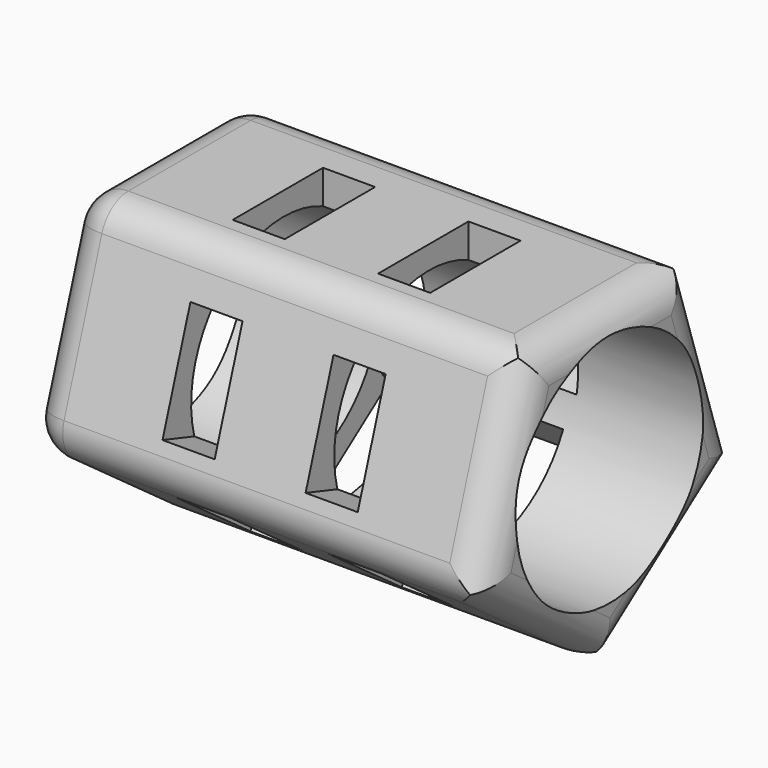
from build123d import *

# Parameters (mm, degrees)
F0_R         = 17.1087851354
F1_DEPTH     = 66.548
F2_T1_DEPTH  = 55.1463138897
F2_T3_DEPTH  = 55.1463138897
F2_T5_DEPTH  = 55.1463138897
F2_T7_DEPTH  = 55.1463138897
F2_T9_DEPTH  = 55.1463138897
F3_T1_DEPTH  = 22.3646418052
F3_T3_DEPTH  = 22.3646418052
F3_T5_DEPTH  = 22.3646418052
F3_T7_DEPTH  = 22.3646418052
F3_T9_DEPTH  = 22.3646418052
F3_T11_DEPTH = 65.6150901057
F3_T16_DEPTH = 5.1816
F3_T22_DEPTH = 5.1816
F3_T28_DEPTH = 5.1816
F3_T34_DEPTH = 5.1816
F3_T40_DEPTH = 5.1816
F4_W         = 7.62
F4_H         = 16.51
F5_DEPTH     = 7.874
F6_W         = 7.62
F6_H         = 16.51
F7_DEPTH     = 7.112
F8_W         = 7.62
F8_H         = 16.51
F9_DEPTH     = 12.192
F10_W        = 7.62
F10_H        = 16.51
F11_DEPTH    = 24.384
F12_W        = 7.62
F12_H        = 16.51
F13_DEPTH    = 25.4


# Not quite as in the source:
# - a fillet or chamfer that OpenCascade refuses, or shapes differently, is made with other operations: its cross-section is extruded or revolved along the edge and cut away or added


with BuildPart() as f1:
    # F0 (on Right) → F1 (new body)
    with BuildSketch(Plane.YZ):
        Polygon((14.8731569449, 20.4711443192), (-14.8731569449, 20.4711443192), (-24.0652734568, -7.8192813413), (0, -25.3037259558), (24.0652734568, -7.8192813413), align=None)
        Circle(F0_R, mode=Mode.SUBTRACT)
    extrude(amount=F1_DEPTH)

    # F2: fillet of radius 5.08 on 5 edges, made by hand

    # F2_s2 → F2_t1 (cut)
    with BuildSketch(Plane(origin=(0, 8.5205740845, 26.2236305872), x_dir=(1, 0, 0), z_dir=(0, -0.3090169944, -0.9510565163))):
        with BuildLine():
            ThreePointArc((61.468, 20.4711443192), (65.0601024484, 18.9832467676), (66.548, 15.3911443192))
            Line((66.548, 15.3911443192), (66.548, 20.4711443192))
            Line((66.548, 20.4711443192), (61.468, 20.4711443192))
        make_face()
    extrude(amount=F2_T1_DEPTH, mode=Mode.SUBTRACT)

    # F2_s4 → F2_t3 (cut)
    with BuildSketch(Plane.XZ.offset(-27.5731569449)):
        with BuildLine():
            ThreePointArc((61.468, 20.4711443192), (65.0601024484, 18.9832467676), (66.548, 15.3911443192))
            Line((66.548, 15.3911443192), (66.548, 20.4711443192))
            Line((66.548, 20.4711443192), (61.468, 20.4711443192))
        make_face()
    extrude(amount=F2_T3_DEPTH, mode=Mode.SUBTRACT)

    # F2_s6 → F2_t5 (cut)
    with BuildSketch(Plane(origin=(0, 8.5205740845, -26.2236305872), x_dir=(1, 0, 0), z_dir=(0, -0.3090169944, 0.9510565163))):
        with BuildLine():
            ThreePointArc((61.468, 20.4711443192), (65.0601024484, 18.9832467676), (66.548, 15.3911443192))
            Line((66.548, 15.3911443192), (66.548, 20.4711443192))
            Line((66.548, 20.4711443192), (61.468, 20.4711443192))
        make_face()
    extrude(amount=F2_T5_DEPTH, mode=Mode.SUBTRACT)

    # F2_s8 → F2_t7 (cut)
    with BuildSketch(Plane(origin=(0, -22.307152557, -16.2070950113), x_dir=(1, 0, 0), z_dir=(0, 0.8090169944, 0.5877852523))):
        with BuildLine():
            ThreePointArc((61.468, 20.4711443192), (65.0601024484, 18.9832467676), (66.548, 15.3911443192))
            Line((66.548, 15.3911443192), (66.548, 20.4711443192))
            Line((66.548, 20.4711443192), (61.468, 20.4711443192))
        make_face()
    extrude(amount=F2_T7_DEPTH, mode=Mode.SUBTRACT)

    # F2_s10 → F2_t9 (cut)
    with BuildSketch(Plane(origin=(0, -22.307152557, 16.2070950113), x_dir=(1, 0, 0), z_dir=(0, 0.8090169944, -0.5877852523))):
        with BuildLine():
            ThreePointArc((61.468, 20.4711443192), (65.0601024484, 18.9832467676), (66.548, 15.3911443192))
            Line((66.548, 15.3911443192), (66.548, 20.4711443192))
            Line((66.548, 20.4711443192), (61.468, 20.4711443192))
        make_face()
    extrude(amount=F2_T9_DEPTH, mode=Mode.SUBTRACT)

    # F3: fillet of radius 5.08 on 14 edges, made by hand

    # F3_s2 → F3_t1 (cut)
    with BuildSketch(Plane(origin=(0, 3.4555271955, -10.6350191617), x_dir=(1, 0, 0), z_dir=(0, -0.3090169944, 0.9510565163))):
        with BuildLine():
            ThreePointArc((5.08, 20.4711443192), (1.4878975516, 18.9832467676), (0, 15.3911443192))
            Line((0, 15.3911443192), (0, 20.4711443192))
            Line((0, 20.4711443192), (5.08, 20.4711443192))
        make_face()
    extrude(amount=F3_T1_DEPTH, mode=Mode.SUBTRACT)

    # F3_s4 → F3_t3 (cut)
    with BuildSketch(Plane.XZ.offset(-11.1823209026)):
        with BuildLine():
            ThreePointArc((0, 15.3911443192), (1.4878975516, 18.9832467676), (5.08, 20.4711443192))
            Line((5.08, 20.4711443192), (0, 20.4711443192))
            Line((0, 20.4711443192), (0, 15.3911443192))
        make_face()
    extrude(amount=F3_T3_DEPTH, mode=Mode.SUBTRACT)

    # F3_s6 → F3_t5 (cut)
    with BuildSketch(Plane(origin=(0, 3.4555271955, 10.6350191617), x_dir=(1, 0, 0), z_dir=(0, -0.3090169944, -0.9510565163))):
        with BuildLine():
            ThreePointArc((0, 15.3911443192), (1.4878975516, 18.9832467676), (5.08, 20.4711443192))
            Line((5.08, 20.4711443192), (0, 20.4711443192))
            Line((0, 20.4711443192), (0, 15.3911443192))
        make_face()
    extrude(amount=F3_T5_DEPTH, mode=Mode.SUBTRACT)

    # F3_s8 → F3_t7 (cut)
    with BuildSketch(Plane(origin=(0, -9.0466876467, 6.5728033129), x_dir=(1, 0, 0), z_dir=(0, 0.8090169944, -0.5877852523))):
        with BuildLine():
            ThreePointArc((0, 15.3911443192), (1.4878975516, 18.9832467676), (5.08, 20.4711443192))
            Line((5.08, 20.4711443192), (0, 20.4711443192))
            Line((0, 20.4711443192), (0, 15.3911443192))
        make_face()
    extrude(amount=F3_T7_DEPTH, mode=Mode.SUBTRACT)

    # F3_s10 → F3_t9 (cut)
    with BuildSketch(Plane(origin=(0, -9.0466876467, -6.5728033129), x_dir=(1, 0, 0), z_dir=(0, 0.8090169944, 0.5877852523))):
        with BuildLine():
            ThreePointArc((0, 15.3911443192), (1.4878975516, 18.9832467676), (5.08, 20.4711443192))
            Line((5.08, 20.4711443192), (0, 20.4711443192))
            Line((0, 20.4711443192), (0, 15.3911443192))
        make_face()
    extrude(amount=F3_T9_DEPTH, mode=Mode.SUBTRACT)

    # F3_s12 → F3_t11 (cut)
    with BuildSketch(Plane.YZ.offset(5.08)):
        with BuildLine():
            ThreePointArc((-22.9247423963, -4.3090876728), (-22.9247423963, -7.4487003356), (-21.0793243751, -9.9887003356))
            Line((-21.0793243751, -9.9887003356), (-24.0652734568, -7.8192813413))
            Line((-24.0652734568, -7.8192813413), (-22.9247423963, -4.3090876728))
        make_face()
        with BuildLine():
            ThreePointArc((-11.1823209026, 20.4711443192), (-14.1682699842, 19.5009506506), (-16.0136880054, 16.9609506506))
            Line((-16.0136880054, 16.9609506506), (-14.8731569449, 20.4711443192))
            Line((-14.8731569449, 20.4711443192), (-11.1823209026, 20.4711443192))
        make_face()
        with BuildLine():
            ThreePointArc((2.9859490816, -23.1343069615), (0, -24.1045006301), (-2.9859490816, -23.1343069615))
            Line((-2.9859490816, -23.1343069615), (0, -25.3037259558))
            Line((0, -25.3037259558), (2.9859490816, -23.1343069615))
        make_face()
        with BuildLine():
            ThreePointArc((22.9247423963, -4.3090876728), (22.9247423963, -7.4487003356), (21.0793243751, -9.9887003356))
            Line((21.0793243751, -9.9887003356), (24.0652734568, -7.8192813413))
            Line((24.0652734568, -7.8192813413), (22.9247423963, -4.3090876728))
        make_face()
        with BuildLine():
            ThreePointArc((16.0136880054, 16.9609506506), (14.1682699842, 19.5009506506), (11.1823209026, 20.4711443192))
            Line((11.1823209026, 20.4711443192), (14.8731569449, 20.4711443192))
            Line((14.8731569449, 20.4711443192), (16.0136880054, 16.9609506506))
        make_face()
    extrude(amount=F3_T11_DEPTH, mode=Mode.SUBTRACT)


with BuildPart() as f3_tool14:
    # F3_s15 → F3_t16 (new body)
    with BuildSketch(Plane.YZ.offset(5.08)):
        Polygon((18.0933752935, -5.8788940042), (21.1390433568, -10.0708964622), (24.18471142, -7.8580890881), (23.0213697383, -4.2776915461), align=None)
    extrude(amount=-F3_T16_DEPTH)

    # F3_s17 → F3_t18 (revolve, cut)
    with BuildSketch(Plane(origin=(5.08, 18.0933752935, -5.8788940042), x_dir=(0, -0.9510565163, 0.3090169944), z_dir=(0, -0.3090169944, -0.9510565163))):
        with BuildLine():
            ThreePointArc((0, -5.08), (5.08, 0), (0, 5.08))
            Line((0, 5.08), (0, -5.08))
        make_face()
    revolve(axis=Axis((5.08, 18.0933752935, -5.8788940042), (-1, 0, 0)), mode=Mode.SUBTRACT)


with BuildPart() as f1_1:
    add(f1.part)

    # F3_t13: cut F3_tool14
    add(f3_tool14.part, mode=Mode.SUBTRACT)


with BuildPart() as f3_tool20:
    # F3_s21 → F3_t22 (new body)
    with BuildSketch(Plane.YZ.offset(5.08)):
        Polygon((11.1823209026, 15.3911443192), (11.1823209026, 20.5727443192), (14.9469736657, 20.5727443192), (16.1103153474, 16.9923467773), align=None)
    extrude(amount=-F3_T22_DEPTH)

    # F3_s23 → F3_t24 (revolve, cut)
    with BuildSketch(Plane(origin=(5.08, 11.1823209026, 15.3911443192), x_dir=(0, -0.5877852523, -0.8090169944), z_dir=(0, 0.8090169944, -0.5877852523))):
        with BuildLine():
            ThreePointArc((0, -5.08), (5.08, 0), (0, 5.08))
            Line((0, 5.08), (0, -5.08))
        make_face()
    revolve(axis=Axis((5.08, 11.1823209026, 15.3911443192), (-1, 0, 0)), mode=Mode.SUBTRACT)


with BuildPart() as f1_2:
    add(f1_1.part)

    # F3_t19: cut F3_tool20
    add(f3_tool20.part, mode=Mode.SUBTRACT)


with BuildPart() as f3_tool26:
    # F3_s27 → F3_t28 (new body)
    with BuildSketch(Plane.YZ.offset(5.08)):
        Polygon((-11.1823209026, 15.3911443192), (-11.1823209026, 20.5727443192), (-14.9469736657, 20.5727443192), (-16.1103153474, 16.9923467773), align=None)
    extrude(amount=-F3_T28_DEPTH)

    # F3_s29 → F3_t30 (revolve, cut)
    with BuildSketch(Plane(origin=(5.08, -11.1823209026, 15.3911443192), x_dir=(0, 0.5877852523, -0.8090169944), z_dir=(0, 0.8090169944, 0.5877852523))):
        with BuildLine():
            ThreePointArc((0, -5.08), (5.08, 0), (0, 5.08))
            Line((0, 5.08), (0, -5.08))
        make_face()
    revolve(axis=Axis((5.08, -11.1823209026, 15.3911443192), (-1, 0, 0)), mode=Mode.SUBTRACT)


with BuildPart() as f1_3:
    add(f1_2.part)

    # F3_t25: cut F3_tool26
    add(f3_tool26.part, mode=Mode.SUBTRACT)


with BuildPart() as f3_tool32:
    # F3_s33 → F3_t34 (new body)
    with BuildSketch(Plane.YZ.offset(5.08)):
        Polygon((-18.0933752935, -5.8788940042), (-23.0213697383, -4.2776915461), (-24.18471142, -7.8580890881), (-21.1390433568, -10.0708964622), align=None)
    extrude(amount=-F3_T34_DEPTH)

    # F3_s35 → F3_t36 (revolve, cut)
    with BuildSketch(Plane(origin=(5.08, -18.0933752935, -5.8788940042), x_dir=(0, 0.9510565163, 0.3090169944), z_dir=(0, -0.3090169944, 0.9510565163))):
        with BuildLine():
            ThreePointArc((0, -5.08), (5.08, 0), (0, 5.08))
            Line((0, 5.08), (0, -5.08))
        make_face()
    revolve(axis=Axis((5.08, -18.0933752935, -5.8788940042), (-1, 0, 0)), mode=Mode.SUBTRACT)


with BuildPart() as f1_4:
    add(f1_3.part)

    # F3_t31: cut F3_tool32
    add(f3_tool32.part, mode=Mode.SUBTRACT)


with BuildPart() as f3_tool38:
    # F3_s39 → F3_t40 (new body)
    with BuildSketch(Plane.YZ.offset(5.08)):
        Polygon((0, -19.0245006301), (3.0456680633, -23.2165030881), (0, -25.4293104623), (-3.0456680633, -23.2165030881), align=None)
    extrude(amount=-F3_T40_DEPTH)

    # F3_s41 → F3_t42 (revolve, cut)
    with BuildSketch(Plane(origin=(5.08, 0, -19.0245006301), x_dir=(0, 0, 1), z_dir=(0, -1, 0))):
        with BuildLine():
            ThreePointArc((0, -5.08), (5.08, 0), (0, 5.08))
            Line((0, 5.08), (0, -5.08))
        make_face()
    revolve(axis=Axis((5.08, 0, -19.0245006301), (-1, 0, 0)), mode=Mode.SUBTRACT)


with BuildPart() as f1_5:
    add(f1_4.part)

    # F3_t37: cut F3_tool38
    add(f3_tool38.part, mode=Mode.SUBTRACT)

    # F4 (on face) → F5 (cut)
    with BuildSketch(Plane(origin=(0, 19.4692152008, 6.3259314889), x_dir=(-1, 0, 0), z_dir=(0, 0.9510565163, 0.3090169944))):
        with Locations((-44.3987917626, 0.1162888882)):
            Rectangle(F4_W, F4_H)
        with Locations((-22.1492082374, 0.1162888882)):
            Rectangle(F4_W, F4_H)
    extrude(amount=-F5_DEPTH, mode=Mode.SUBTRACT)

    # F6 (on face) → F7 (cut)
    with BuildSketch(Plane(origin=(0, 12.0326367284, -16.5615036486), x_dir=(1, 0, 0), z_dir=(0, 0.5877852523, -0.8090169944))):
        with Locations((23.0322839265, 0.0248623613)):
            Rectangle(F6_W, F6_H)
        with Locations((43.5157160735, 0.0248623613)):
            Rectangle(F6_W, F6_H)
    extrude(amount=-F7_DEPTH, mode=Mode.SUBTRACT)

    # F8 (on face) → F9 (cut)
    with BuildSketch(Plane.XY.offset(20.4711443192)):
        with Locations((22.6449199492, -1.054919551)):
            Rectangle(F8_W, F8_H)
        with Locations((43.9030800508, -1.054919551)):
            Rectangle(F8_W, F8_H)
    extrude(amount=-F9_DEPTH, mode=Mode.SUBTRACT)

    # F10 (on face) → F11 (cut)
    with BuildSketch(Plane(origin=(0, -19.4692152008, 6.3259314889), x_dir=(1, 0, 0), z_dir=(0, -0.9510565163, 0.3090169944))):
        with Locations((22.8148490661, -1.0384099957)):
            Rectangle(F10_W, F10_H)
        with Locations((43.7331509339, -1.0384099957)):
            Rectangle(F10_W, F10_H)
    extrude(amount=-F11_DEPTH, mode=Mode.SUBTRACT)

    # F12 (on face) → F13 (cut)
    with BuildSketch(Plane(origin=(0, -12.0326367284, -16.5615036486), x_dir=(1, 0, 0), z_dir=(0, -0.5877852523, -0.8090169944))):
        with Locations((22.2020648891, 0.2502023774)):
            Rectangle(F12_W, F12_H)
        with Locations((44.3459351109, 0.2502023774)):
            Rectangle(F12_W, F12_H)
    extrude(amount=-F13_DEPTH, mode=Mode.SUBTRACT)


solid = f1_5.part
